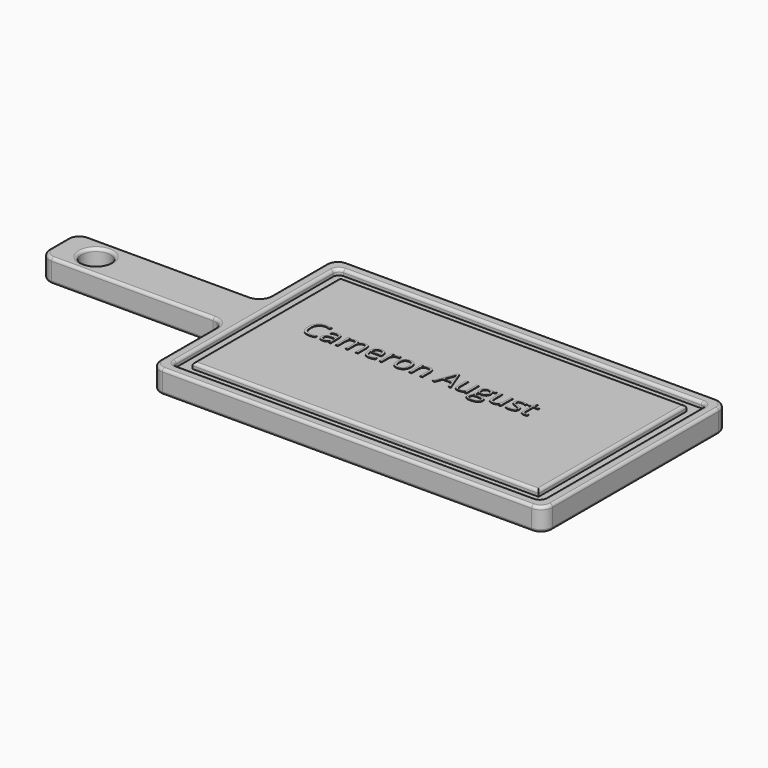
from build123d import *

# Parameters (mm, degrees)
F0_W         = 203.2
F0_H         = 50.8
F1_DEPTH     = 25.4
F2_R         = 15.875
F3_DEPTH     = 25.4
F5_DEPTH     = 6.35
F6_R         = 6.35
F7_R         = 12.7
F8_R         = 3.175
F9_TEXT_SIZE = 32.3721523021
F10_DEPTH    = 0.508


# Not quite as in the source:
# - Text() gives the source's letters only with a copy of the font that has no kerning and outlines rounded to 1/6400 em; it was checked with that copy


with BuildPart() as f1:
    # F0 (on Top) → F1 (new body)
    with BuildSketch(Plane.XY):
        with Locations((-101.6, 127)):
            Rectangle(F0_W, F0_H)
        Polygon((0, 101.6), (0, 0), (431.8, 0), (431.8, 254), (0, 254), (0, 152.4), align=None)
    extrude(amount=F1_DEPTH)

    # F2 (on face) → F3 (cut)
    with BuildSketch(Plane.XY.offset(25.4)):
        with Locations((-161.925, 127)):
            Circle(F2_R)
    extrude(amount=-F3_DEPTH, mode=Mode.SUBTRACT)

    # F4 (on face) → F5 (cut)
    with BuildSketch(Plane.XY.offset(25.4)):
        Polygon((12.6999982595, 101.6), (12.6999982595, 12.6999982595), (419.1000017405, 12.6999982595), (419.1000017405, 241.3000017405), (12.6999982595, 241.3000017405), (12.6999982595, 152.4), align=None)
        Polygon((406.3999953747, 25.4000046253), (25.4000046253, 25.4000046253), (25.4000046253, 101.6), (25.4000046253, 152.4), (25.4000046253, 228.5999953747), (406.3999953747, 228.5999953747), align=None, mode=Mode.SUBTRACT)
    extrude(amount=-F5_DEPTH, mode=Mode.SUBTRACT)

    # F6
    f6_edges = [f1.edges().sort_by_distance(p)[0] for p in [
        (12.699998, 241.300002, 22.225),
        (419.100002, 12.699998, 22.225),
        (419.100002, 241.300002, 22.225),
        (12.699998, 12.699998, 22.225),
    ]]
    fillet(f6_edges, radius=F6_R)

    # F7
    f7_edges = [f1.edges().sort_by_distance(p)[0] for p in [
        (0, 152.4, 12.7),
        (0, 101.6, 12.7),
        (0, 254, 12.7),
        (0, 0, 12.7),
        (-203.2, 101.6, 12.7),
        (-203.2, 152.4, 12.7),
        (431.8, 0, 12.7),
        (431.8, 254, 12.7),
    ]]
    fillet(f7_edges, radius=F7_R)

    # F8
    f8_edges = [f1.edges().sort_by_distance(p)[0] for p in [
        (406.399995, 127, 25.4),
        (215.9, 25.400005, 25.4),
        (25.400005, 127, 25.4),
        (215.9, 228.599995, 25.4),
        (-101.6, 101.6, 25.4),
        (-199.480256, 105.319744, 25.4),
        (-3.719744, 97.880256, 25.4),
        (-203.2, 127, 25.4),
        (0, 50.8, 25.4),
        (-199.480256, 148.680256, 25.4),
        (3.719744, 3.719744, 25.4),
        (-101.6, 152.4, 25.4),
        (215.9, 0, 25.4),
        (-3.719744, 156.119744, 25.4),
        (428.080256, 3.719744, 25.4),
        (0, 203.2, 25.4),
        (431.8, 127, 25.4),
        (3.719744, 250.280256, 25.4),
        (428.080256, 250.280256, 25.4),
        (215.9, 254, 25.4),
        (215.9, 12.699998, 25.4),
        (14.55987, 14.55987, 25.4),
        (417.24013, 14.55987, 25.4),
        (12.699998, 127, 25.4),
        (419.100002, 127, 25.4),
        (14.55987, 239.44013, 25.4),
        (417.24013, 239.44013, 25.4),
        (215.9, 241.300002, 25.4),
        (-177.8, 127, 25.4),
        (-101.6, 101.6, 0),
        (-199.480256, 105.319744, 0),
        (-3.719744, 97.880256, 0),
        (-203.2, 127, 0),
        (0, 50.8, 0),
        (-199.480256, 148.680256, 0),
        (3.719744, 3.719744, 0),
        (-101.6, 152.4, 0),
        (215.9, 0, 0),
        (-3.719744, 156.119744, 0),
        (428.080256, 3.719744, 0),
        (0, 203.2, 0),
        (431.8, 127, 0),
        (3.719744, 250.280256, 0),
        (428.080256, 250.280256, 0),
        (215.9, 254, 0),
        (-177.8, 127, 0),
    ]]
    fillet(f8_edges, radius=F8_R)

    # F9 (on face) → F10 (join)
    with BuildSketch(Plane.XY.offset(25.4)):
        with Locations((60.3249982595, 127.0000046253)):
            Text('Cameron August', F9_TEXT_SIZE, font='Open Sans', text_align=(TextAlign.LEFT, TextAlign.BOTTOM))
    extrude(amount=F10_DEPTH)


solid = f1.part
